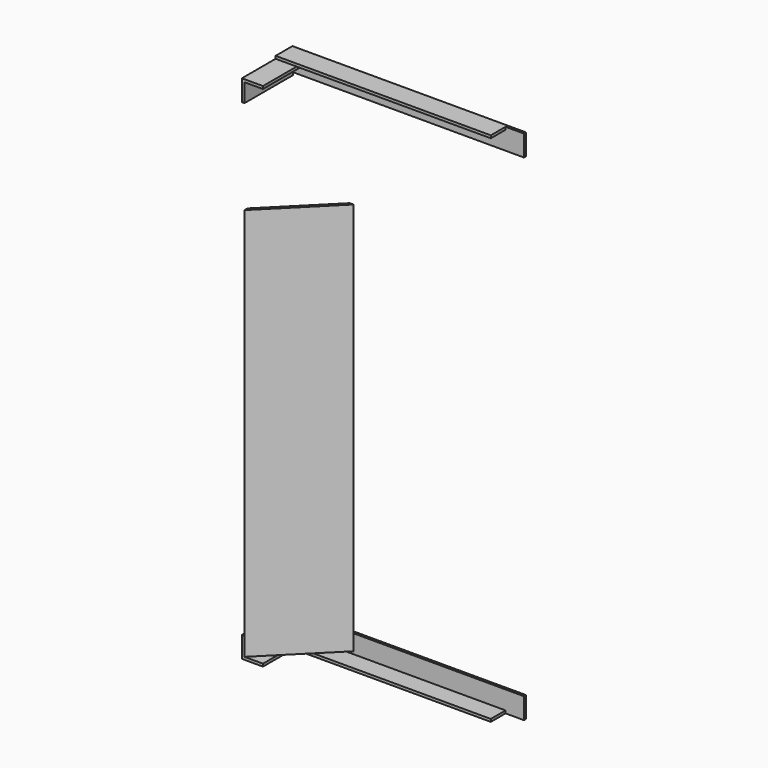
from build123d import *

# Parameters (mm, degrees)
F0_W      = 22.225
F0_H      = 22.225
F0_W_2    = 3.175
F0_H_2    = 3.175
F1_DEPTH  = 3.175
F2_START  = 3.175
F2_DEPTH  = 474.218
F3_DEPTH  = 22.225
F4_START  = -619.50092
F1_FACE_W = 76.2
F1_FACE_H = 25.4
F4_DEPTH  = 3.175
F5_START  = 571.87592
F3_FACE_W = 76.2
F3_FACE_H = 3.175
F5_DEPTH  = 22.225
F6_DEPTH  = 3.175
F7_DEPTH  = 25.4
F8_START  = 565.52592
F7_FACE_W = 3.175
F7_FACE_H = 73.025
F8_DEPTH  = 25.4
F9_START  = 609.97592
F6_FACE_W = 22.225
F6_FACE_H = 73.025
F9_DEPTH  = 3.175
F10_W     = 3.175
F10_H     = 3.175
F10_H_2   = 22.225
F11_DEPTH = 205.54188
F12_DEPTH = 183.31688
F13_DEPTH = 205.54188
F10_W_2   = 22.225
F14_DEPTH = 183.31688


with BuildPart() as f1:
    # F0 (on Top) → F1 (new body)
    with BuildSketch(Plane.XY):
        Polygon((38.1, 50.8), (38.1, 73.025), (15.875, 50.8), align=None)
        Polygon((15.875, 50.8), (38.1, 73.025), (33.6098719395, 73.025), (11.3848719395, 50.8), align=None)
        Polygon((33.6098719395, 73.025), (-12.7, 73.025), (-12.7, 50.8), (11.3848719395, 50.8), align=None)
        with Locations((-23.8125, 61.9125)):
            Rectangle(F0_W, F0_H)
        with Locations((-36.5125, 61.9125)):
            Rectangle(F0_W_2, F0_H)
        Polygon((38.1, 76.2), (-34.925, 76.2), (-34.925, 73.025), (-12.7, 73.025), (33.6098719395, 73.025), (38.1, 73.025), align=None)
        with Locations((-36.5125, 74.6125)):
            Rectangle(F0_W_2, F0_H_2)
    extrude(amount=-F1_DEPTH)

    # F0 (on Top) → F3 (join)
    with BuildSketch(Plane.XY):
        Polygon((38.1, 76.2), (-34.925, 76.2), (-34.925, 73.025), (-12.7, 73.025), (33.6098719395, 73.025), (38.1, 73.025), align=None)
        with Locations((-36.5125, 74.6125)):
            Rectangle(F0_W_2, F0_H_2)
    extrude(amount=F3_DEPTH)

    # F10 (on face) → F11 (join)
    with BuildSketch(Plane.YZ.offset(38.1)):
        with Locations((74.6125, -1.5875)):
            Rectangle(F10_W, F10_H)
        with Locations((74.6125, 11.1125)):
            Rectangle(F10_W, F10_H_2)
    extrude(amount=F11_DEPTH)

    # F12 (add): a face of the model
    f12_faces = [f1.faces().sort_by_distance(p)[0] for p in [
        (38.1, 61.9125, -1.5875),
    ]]
    extrude(f12_faces, amount=F12_DEPTH)


with BuildPart() as f2:
    # F0 (on Top) → F2 (new body)
    with BuildSketch(Plane.XY.offset(F2_START)):
        Polygon((15.875, 50.8), (38.1, 73.025), (33.6098719395, 73.025), (11.3848719395, 50.8), align=None)
        Polygon((-12.7, 22.225), (15.875, 50.8), (11.3848719395, 50.8), (-12.7, 26.7151280605), align=None)
        Polygon((-12.7, 26.7151280605), (-34.925, 4.4901280605), (-34.925, 0), (-12.7, 22.225), align=None)
    extrude(amount=F2_DEPTH)


with BuildPart() as f4:
    # F1_face (on face) → F4 (new body)
    with BuildSketch(Plane(origin=(0, 63.5, -3.175), x_dir=(1, 0, 0), z_dir=(0, 0, -1)).offset(F4_START)):
        Rectangle(F1_FACE_W, F1_FACE_H)
    extrude(amount=-F4_DEPTH)

    # F3_face (on face) → F5 (join)
    with BuildSketch(Plane(origin=(0, 74.6125, 22.225), x_dir=(1, 0, 0), z_dir=(0, 0, 1)).offset(F5_START)):
        Rectangle(F3_FACE_W, F3_FACE_H)
    extrude(amount=F5_DEPTH)

    # F10 (on face) → F13 (join)
    with BuildSketch(Plane.YZ.offset(38.1)):
        with Locations((74.6125, 605.21342)):
            Rectangle(F10_W, F10_H_2)
        with Locations((74.6125, 617.91342)):
            Rectangle(F10_W, F10_H)
    extrude(amount=F13_DEPTH)

    # F10 (on face) → F14 (join)
    with BuildSketch(Plane.YZ.offset(38.1)):
        with Locations((61.9125, 617.91342)):
            Rectangle(F10_W_2, F10_H)
    extrude(amount=F14_DEPTH)


with BuildPart() as f6:
    # F0 (on Top) → F6 (new body)
    with BuildSketch(Plane.XY):
        Polygon((-12.7, 0), (-12.7, 22.225), (-34.925, 0), align=None)
        Polygon((-12.7, 26.7151280605), (-34.925, 4.4901280605), (-34.925, 0), (-12.7, 22.225), align=None)
        Polygon((-12.7, 50.8), (-34.925, 50.8), (-34.925, 47.625), (-34.925, 4.4901280605), (-12.7, 26.7151280605), align=None)
        with Locations((-23.8125, 61.9125)):
            Rectangle(F0_W, F0_H)
    extrude(amount=F6_DEPTH)

    # F0 (on Top) → F7 (join)
    with BuildSketch(Plane.XY):
        Polygon((-34.925, 47.625), (-38.1, 47.625), (-38.1, 0), (-34.925, 0), (-34.925, 4.4901280605), align=None)
        with Locations((-36.5125, 61.9125)):
            Rectangle(F0_W_2, F0_H)
        with Locations((-36.5125, 49.2125)):
            Rectangle(F0_W_2, F0_H_2)
    extrude(amount=F7_DEPTH)


with BuildPart() as f8:
    # F7_face (on face) → F8 (new body)
    with BuildSketch(Plane(origin=(-36.5125, 36.5125, 25.4), x_dir=(1, 0, 0), z_dir=(0, 0, 1)).offset(F8_START)):
        Rectangle(F7_FACE_W, F7_FACE_H)
    extrude(amount=F8_DEPTH)

    # F6_face (on face) → F9 (join)
    with BuildSketch(Plane(origin=(-23.8125, 36.5125, 3.175), x_dir=(1, 0, 0), z_dir=(0, 0, 1)).offset(F9_START)):
        Rectangle(F6_FACE_W, F6_FACE_H)
    extrude(amount=F9_DEPTH)


solid = Compound([f1.part, f2.part, f4.part, f6.part, f8.part])
